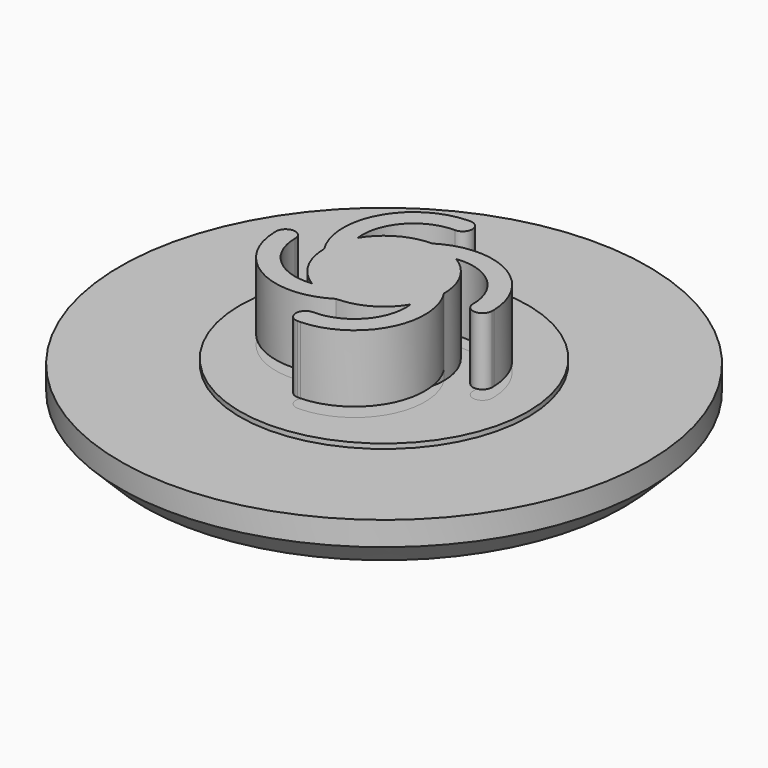
from build123d import *
from build123d import SkipClean  # not in build123d's __all__

# Parameters (mm, degrees)
F0_R     = 11
F1_DEPTH = 2
F2_SIZE  = 1
F3_R     = 6
F4_DEPTH = 0.2
F6_DEPTH = 3.2
F7_DEPTH = 0.4


with BuildPart() as f1:
    # F0 (on Top) → F1 (new body)
    with BuildSketch(Plane.XY):
        Circle(F0_R)
    extrude(amount=F1_DEPTH)

    # F2
    f2_edges = [f1.edges().sort_by_distance(p)[0] for p in [
        (-11, 0, 0),
    ]]
    chamfer(f2_edges, length=F2_SIZE)

    # F3 (on face) → F4 (join)
    with BuildSketch(Plane.XY.offset(2)):
        Circle(F3_R)
    extrude(amount=F4_DEPTH)

    # F5 (on face) → F6 (join)
    with BuildSketch(Plane.XY.offset(2.2)):
        with BuildLine():
            ThreePointArc((-0.0052788349, 3.7000174165), (0.3973518743, 4.0973692908), (0, 4.5))
            ThreePointArc((0, 4.5), (-0.0556126102, 4.4996563466), (-0.1112167263, 4.4986254389))
            ThreePointArc((-0.1112167263, 4.4986254389), (-2.6104676107, 2.9421967987), (-2.5, 0))
            ThreePointArc((-2.5, 0), (-2.4073466074, 0.6743013511), (-2.1362541503, 1.2986216559))
            ThreePointArc((-2.1362541503, 1.2986216559), (-1.6153328632, 2.9825624536), (-0.0052788349, 3.7000174165))
        make_face()
        with BuildLine():
            ThreePointArc((3.7000174165, 0.0052788349), (4.0973692908, -0.3973518743), (4.5, 0))
            ThreePointArc((4.5, 0), (4.4996563466, 0.0556126102), (4.4986254389, 0.1112167263))
            ThreePointArc((4.4986254389, 0.1112167263), (2.9421967987, 2.6104676107), (0, 2.5))
            ThreePointArc((0, 2.5), (0.6743013511, 2.4073466074), (1.2986216559, 2.1362541503))
            ThreePointArc((1.2986216559, 2.1362541503), (2.9825624536, 1.6153328632), (3.7000174165, 0.0052788349))
        make_face()
        with BuildLine():
            ThreePointArc((0, -4.5), (0.0556126102, -4.4996563466), (0.1112167263, -4.4986254389))
            ThreePointArc((0.1112167263, -4.4986254389), (2.6104676107, -2.9421967987), (2.5, 0))
            ThreePointArc((2.5, 0), (2.4073466074, -0.6743013511), (2.1362541503, -1.2986216559))
            ThreePointArc((2.1362541503, -1.2986216559), (1.6153328632, -2.9825624536), (0.0052788349, -3.7000174165))
            ThreePointArc((0.0052788349, -3.7000174165), (-0.3973518743, -4.0973692908), (0, -4.5))
        make_face()
        with BuildLine():
            ThreePointArc((-4.5, 0), (-4.4996563466, -0.0556126102), (-4.4986254389, -0.1112167263))
            ThreePointArc((-4.4986254389, -0.1112167263), (-2.9421967987, -2.6104676107), (0, -2.5))
            ThreePointArc((0, -2.5), (-0.6743013511, -2.4073466074), (-1.2986216559, -2.1362541503))
            ThreePointArc((-1.2986216559, -2.1362541503), (-2.9825624536, -1.6153328632), (-3.7000174165, -0.0052788349))
            ThreePointArc((-3.7000174165, -0.0052788349), (-4.0973692908, 0.3973518743), (-4.5, 0))
        make_face()
        with BuildLine():
            ThreePointArc((1.2986216559, 2.1362541503), (0.6743013511, 2.4073466074), (0, 2.5))
            ThreePointArc((0, 2.5), (-1.2254480528, 2.1790541686), (-2.1362541503, 1.2986216559))
            ThreePointArc((-2.1362541503, 1.2986216559), (-2.4073466074, 0.6743013511), (-2.5, 0))
            ThreePointArc((-2.5, 0), (-2.1790541686, -1.2254480528), (-1.2986216559, -2.1362541503))
            ThreePointArc((-1.2986216559, -2.1362541503), (-0.6743013511, -2.4073466074), (0, -2.5))
            ThreePointArc((0, -2.5), (1.2254480528, -2.1790541686), (2.1362541503, -1.2986216559))
            ThreePointArc((2.1362541503, -1.2986216559), (2.4073466074, -0.6743013511), (2.5, 0))
            ThreePointArc((2.5, 0), (2.1790541686, 1.2254480528), (1.2986216559, 2.1362541503))
        make_face()
    extrude(amount=F6_DEPTH)

    # F5 (on face) → F7 (cut)
    with BuildSketch(Plane.XY.offset(2.2)):
        with BuildLine():
            ThreePointArc((-4.5, 0), (-4.4996563466, -0.0556126102), (-4.4986254389, -0.1112167263))
            ThreePointArc((-4.4986254389, -0.1112167263), (-2.9421967987, -2.6104676107), (0, -2.5))
            ThreePointArc((0, -2.5), (-0.6743013511, -2.4073466074), (-1.2986216559, -2.1362541503))
            ThreePointArc((-1.2986216559, -2.1362541503), (-2.9825624536, -1.6153328632), (-3.7000174165, -0.0052788349))
            ThreePointArc((-3.7000174165, -0.0052788349), (-4.0973692908, 0.3973518743), (-4.5, 0))
        make_face()
        with BuildLine():
            ThreePointArc((-0.0052788349, 3.7000174165), (0.3973518743, 4.0973692908), (0, 4.5))
            ThreePointArc((0, 4.5), (-0.0556126102, 4.4996563466), (-0.1112167263, 4.4986254389))
            ThreePointArc((-0.1112167263, 4.4986254389), (-2.6104676107, 2.9421967987), (-2.5, 0))
            ThreePointArc((-2.5, 0), (-2.4073466074, 0.6743013511), (-2.1362541503, 1.2986216559))
            ThreePointArc((-2.1362541503, 1.2986216559), (-1.6153328632, 2.9825624536), (-0.0052788349, 3.7000174165))
        make_face()
        with BuildLine():
            ThreePointArc((3.7000174165, 0.0052788349), (4.0973692908, -0.3973518743), (4.5, 0))
            ThreePointArc((4.5, 0), (4.4996563466, 0.0556126102), (4.4986254389, 0.1112167263))
            ThreePointArc((4.4986254389, 0.1112167263), (2.9421967987, 2.6104676107), (0, 2.5))
            ThreePointArc((0, 2.5), (0.6743013511, 2.4073466074), (1.2986216559, 2.1362541503))
            ThreePointArc((1.2986216559, 2.1362541503), (2.9825624536, 1.6153328632), (3.7000174165, 0.0052788349))
        make_face()
        with BuildLine():
            ThreePointArc((0, -4.5), (0.0556126102, -4.4996563466), (0.1112167263, -4.4986254389))
            ThreePointArc((0.1112167263, -4.4986254389), (2.6104676107, -2.9421967987), (2.5, 0))
            ThreePointArc((2.5, 0), (2.4073466074, -0.6743013511), (2.1362541503, -1.2986216559))
            ThreePointArc((2.1362541503, -1.2986216559), (1.6153328632, -2.9825624536), (0.0052788349, -3.7000174165))
            ThreePointArc((0.0052788349, -3.7000174165), (-0.3973518743, -4.0973692908), (0, -4.5))
        make_face()
    with SkipClean():  # cleaning this boolean's faces spoils the solid; the shape is the same uncleaned
        extrude(amount=F7_DEPTH, mode=Mode.SUBTRACT)


solid = f1.part
